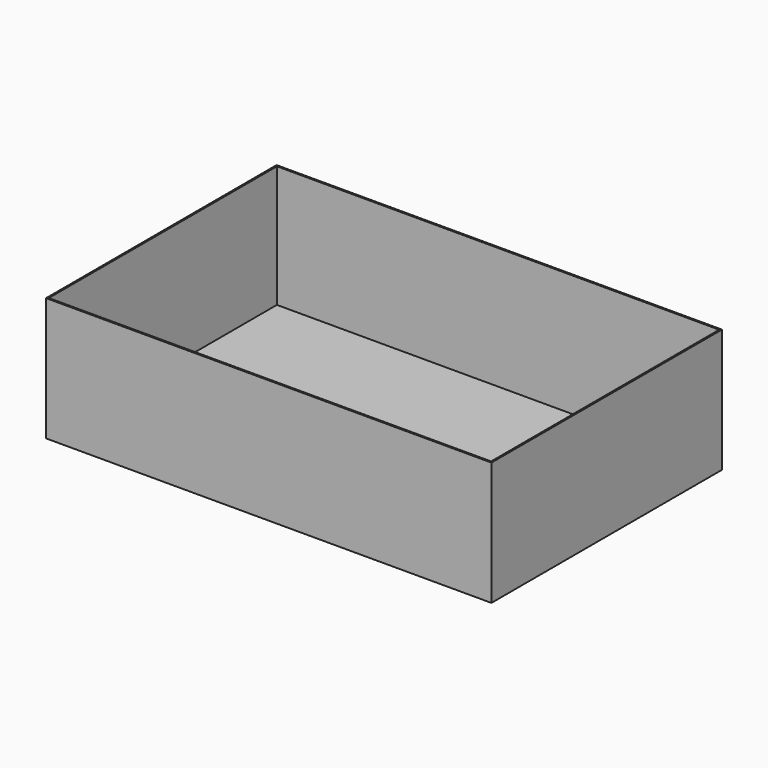
from build123d import *

# Parameters (mm, degrees)
F1_W     = 595
F1_H     = 385
F2_DEPTH = 2
F3_W     = 595
F3_H     = 385
F3_W_2   = 591
F3_H_2   = 381
F4_DEPTH = 163


with BuildPart() as f2:
    # F1 (on Top) → F2 (new body)
    with BuildSketch(Plane.XY):
        with Locations((297.5, -192.5)):
            Rectangle(F1_W, F1_H)
    extrude(amount=F2_DEPTH)

    # F3 (on face) → F4 (join)
    with BuildSketch(Plane.XY.offset(2)):
        with Locations((297.5, -192.5)):
            Rectangle(F3_W, F3_H)
        with Locations((297.5, -192.5)):
            Rectangle(F3_W_2, F3_H_2, mode=Mode.SUBTRACT)
    extrude(amount=F4_DEPTH)


solid = f2.part
